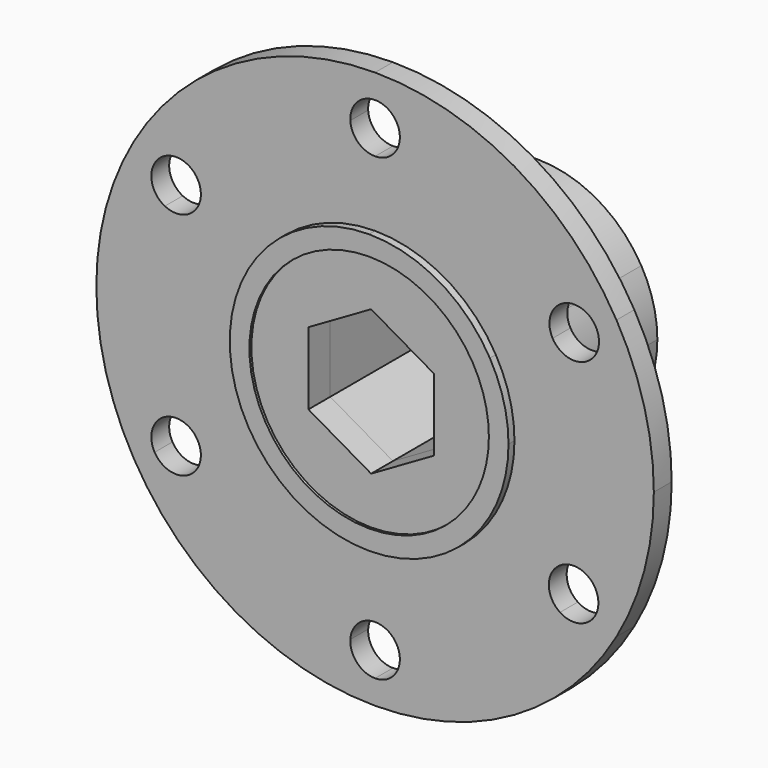
from build123d import *

# Parameters (mm, degrees)
F1_DEPTH = 18.542
F2_DEPTH = 3.048
F3_DEPTH = 2.286
F4_DEPTH = 2.286
F6_DEPTH = 2.794


# Not quite as in the source:
# - a feature of the source that left no trace in its solid (it failed there, or was rolled back) is left out


with BuildPart() as f1:
    # F0 (on Front) → F1 (new body)
    with BuildSketch(Plane.XZ):
        with BuildLine():
            Line((6.4262, 3.7101682999), (10.6292995539, 6.1368289587))
            ThreePointArc((10.6292995539, 6.1368289587), (6.1368289587, 10.6292995539), (0, 12.2736579174))
            Line((0, 12.2736579174), (0, 7.4203365997))
            Line((0, 7.4203365997), (6.4262, 3.7101682999))
        make_face()
        with BuildLine():
            ThreePointArc((12.2736579174, 0), (11.8554431655, 3.1766564221), (10.6292995539, 6.1368289587))
            Line((10.6292995539, 6.1368289587), (6.4262, 3.7101682999))
            Line((6.4262, 3.7101682999), (6.4262, -2.8670745859))
            Line((6.4262, -2.8670745859), (6.4262, -3.7101682999))
            Line((6.4262, -3.7101682999), (10.6292995539, -6.1368289587))
            ThreePointArc((10.6292995539, -6.1368289587), (11.8554431655, -3.1766564221), (12.2736579174, 0))
        make_face()
        with BuildLine():
            ThreePointArc((0, -12.2736579174), (6.1368289587, -10.6292995539), (10.6292995539, -6.1368289587))
            Line((10.6292995539, -6.1368289587), (6.4262, -3.7101682999))
            Line((6.4262, -3.7101682999), (0, -7.4203365997))
            Line((0, -7.4203365997), (0, -12.2736579174))
        make_face()
        with BuildLine():
            Line((0, 7.4203365997), (0, 12.2736579174))
            ThreePointArc((0, 12.2736579174), (-6.1368289587, 10.6292995539), (-10.6292995539, 6.1368289587))
            Line((-10.6292995539, 6.1368289587), (-6.4262, 3.7101682999))
            Line((-6.4262, 3.7101682999), (0, 7.4203365997))
        make_face()
        with BuildLine():
            ThreePointArc((-10.6292995539, -6.1368289587), (-6.1368289587, -10.6292995539), (0, -12.2736579174))
            Line((0, -12.2736579174), (0, -7.4203365997))
            Line((0, -7.4203365997), (-6.4262, -3.7101682999))
            Line((-6.4262, -3.7101682999), (-10.6292995539, -6.1368289587))
        make_face()
        with BuildLine():
            Line((-6.4262, 3.7101682999), (-10.6292995539, 6.1368289587))
            ThreePointArc((-10.6292995539, 6.1368289587), (-12.2736579174, 0), (-10.6292995539, -6.1368289587))
            Line((-10.6292995539, -6.1368289587), (-6.4262, -3.7101682999))
            Line((-6.4262, -3.7101682999), (-6.4262, 3.7101682999))
        make_face()
    extrude(amount=-F1_DEPTH)

    # F0 (on Front) → F6 (join)
    with BuildSketch(Plane.XZ):
        with BuildLine():
            Line((6.4262, 3.7101682999), (10.6292995539, 6.1368289587))
            ThreePointArc((10.6292995539, 6.1368289587), (6.1368289587, 10.6292995539), (0, 12.2736579174))
            Line((0, 12.2736579174), (0, 7.4203365997))
            Line((0, 7.4203365997), (6.4262, 3.7101682999))
        make_face()
        with BuildLine():
            ThreePointArc((12.2736579174, 0), (11.8554431655, 3.1766564221), (10.6292995539, 6.1368289587))
            Line((10.6292995539, 6.1368289587), (6.4262, 3.7101682999))
            Line((6.4262, 3.7101682999), (6.4262, -2.8670745859))
            Line((6.4262, -2.8670745859), (6.4262, -3.7101682999))
            Line((6.4262, -3.7101682999), (10.6292995539, -6.1368289587))
            ThreePointArc((10.6292995539, -6.1368289587), (11.8554431655, -3.1766564221), (12.2736579174, 0))
        make_face()
        with BuildLine():
            ThreePointArc((0, -12.2736579174), (6.1368289587, -10.6292995539), (10.6292995539, -6.1368289587))
            Line((10.6292995539, -6.1368289587), (6.4262, -3.7101682999))
            Line((6.4262, -3.7101682999), (0, -7.4203365997))
            Line((0, -7.4203365997), (0, -12.2736579174))
        make_face()
        with BuildLine():
            Line((0, 7.4203365997), (0, 12.2736579174))
            ThreePointArc((0, 12.2736579174), (-6.1368289587, 10.6292995539), (-10.6292995539, 6.1368289587))
            Line((-10.6292995539, 6.1368289587), (-6.4262, 3.7101682999))
            Line((-6.4262, 3.7101682999), (0, 7.4203365997))
        make_face()
        with BuildLine():
            ThreePointArc((-10.6292995539, -6.1368289587), (-6.1368289587, -10.6292995539), (0, -12.2736579174))
            Line((0, -12.2736579174), (0, -7.4203365997))
            Line((0, -7.4203365997), (-6.4262, -3.7101682999))
            Line((-6.4262, -3.7101682999), (-10.6292995539, -6.1368289587))
        make_face()
        with BuildLine():
            Line((-6.4262, 3.7101682999), (-10.6292995539, 6.1368289587))
            ThreePointArc((-10.6292995539, 6.1368289587), (-12.2736579174, 0), (-10.6292995539, -6.1368289587))
            Line((-10.6292995539, -6.1368289587), (-6.4262, -3.7101682999))
            Line((-6.4262, -3.7101682999), (-6.4262, 3.7101682999))
        make_face()
    extrude(amount=F6_DEPTH)


with BuildPart() as f2:
    # F0 (on Front) → F2 (new body)
    with BuildSketch(Plane.XZ):
        with BuildLine():
            ThreePointArc((0, -14.2875), (7.14375, -12.3733379566), (12.3733379566, -7.14375))
            Line((12.3733379566, -7.14375), (10.6292995539, -6.1368289587))
            ThreePointArc((10.6292995539, -6.1368289587), (6.1368289587, -10.6292995539), (0, -12.2736579174))
            Line((0, -12.2736579174), (0, -14.2875))
        make_face()
        with BuildLine():
            ThreePointArc((-12.3733379566, -7.14375), (-7.14375, -12.3733379566), (0, -14.2875))
            Line((0, -14.2875), (0, -12.2736579174))
            ThreePointArc((0, -12.2736579174), (-6.1368289587, -10.6292995539), (-10.6292995539, -6.1368289587))
            Line((-10.6292995539, -6.1368289587), (-12.3733379566, -7.14375))
        make_face()
        with BuildLine():
            Line((-10.6292995539, 6.1368289587), (-12.3733379566, 7.14375))
            ThreePointArc((-12.3733379566, 7.14375), (-14.2875, 0), (-12.3733379566, -7.14375))
            Line((-12.3733379566, -7.14375), (-10.6292995539, -6.1368289587))
            ThreePointArc((-10.6292995539, -6.1368289587), (-12.2736579174, 0), (-10.6292995539, 6.1368289587))
        make_face()
        with BuildLine():
            Line((0, 12.2736579174), (0, 14.2875))
            ThreePointArc((0, 14.2875), (-7.14375, 12.3733379566), (-12.3733379566, 7.14375))
            Line((-12.3733379566, 7.14375), (-10.6292995539, 6.1368289587))
            ThreePointArc((-10.6292995539, 6.1368289587), (-6.1368289587, 10.6292995539), (0, 12.2736579174))
        make_face()
        with BuildLine():
            Line((10.6292995539, 6.1368289587), (12.3733379566, 7.14375))
            ThreePointArc((12.3733379566, 7.14375), (7.14375, 12.3733379566), (0, 14.2875))
            Line((0, 14.2875), (0, 12.2736579174))
            ThreePointArc((0, 12.2736579174), (6.1368289587, 10.6292995539), (10.6292995539, 6.1368289587))
        make_face()
        with BuildLine():
            ThreePointArc((14.2875, 0), (13.8006652431, 3.6978771069), (12.3733379566, 7.14375))
            Line((12.3733379566, 7.14375), (10.6292995539, 6.1368289587))
            ThreePointArc((10.6292995539, 6.1368289587), (11.8554431655, 3.1766564221), (12.2736579174, 0))
            ThreePointArc((12.2736579174, 0), (11.8554431655, -3.1766564221), (10.6292995539, -6.1368289587))
            Line((10.6292995539, -6.1368289587), (12.3733379566, -7.14375))
            ThreePointArc((12.3733379566, -7.14375), (13.8006652431, -3.6978771069), (14.2875, 0))
        make_face()
    extrude(amount=F2_DEPTH)

    # F0 (on Front) → F3 (join)
    with BuildSketch(Plane.XZ):
        with BuildLine():
            ThreePointArc((2.5363048132, -23.415995125), (11.7362040327, -20.4206558343), (18.9556707318, -13.9794211936))
            ThreePointArc((18.9556707318, -13.9794211936), (17.8690577157, -12.3976727234), (18.1990671233, -10.5072363026))
            Line((18.1990671233, -10.5072363026), (12.3733379566, -7.14375))
            ThreePointArc((12.3733379566, -7.14375), (7.14375, -12.3733379566), (0, -14.2875))
            Line((0, -14.2875), (0, -21.0129545875))
            ThreePointArc((0, -21.0129545875), (1.7469577793, -21.7091166019), (2.5363048132, -23.415995125))
        make_face()
        with BuildLine():
            ThreePointArc((-19.0106942266, -13.9045019625), (-11.7764772938, -20.397457007), (-2.5363048132, -23.415995125))
            ThreePointArc((-2.5363048132, -23.415995125), (-1.7469577793, -21.7091166019), (0, -21.0129545875))
            Line((0, -21.0129545875), (0, -14.2875))
            ThreePointArc((0, -14.2875), (-7.14375, -12.3733379566), (-12.3733379566, -7.14375))
            Line((-12.3733379566, -7.14375), (-18.1977524814, -10.5064772938))
            ThreePointArc((-18.1977524814, -10.5064772938), (-17.9440054082, -11.1190769192), (-17.857457007, -11.7764772938))
            ThreePointArc((-17.857457007, -11.7764772938), (-18.1643003329, -12.9866885434), (-19.0106942266, -13.9045019625))
        make_face()
        with BuildLine():
            ThreePointArc((-18.1977524814, 10.5064772938), (-19.6741253606, 9.3416484847), (-21.5469990398, 9.5114931625))
            ThreePointArc((-21.5469990398, 9.5114931625), (-23.5529545875, 0), (-21.5469990398, -9.5114931625))
            ThreePointArc((-21.5469990398, -9.5114931625), (-19.6741253606, -9.3416484847), (-18.1977524814, -10.5064772938))
            Line((-18.1977524814, -10.5064772938), (-12.3733379566, -7.14375))
            ThreePointArc((-12.3733379566, -7.14375), (-14.2875, 0), (-12.3733379566, 7.14375))
            Line((-12.3733379566, 7.14375), (-18.1977524814, 10.5064772938))
        make_face()
        with BuildLine():
            ThreePointArc((0, 21.0129545875), (-1.7469577793, 21.7091166019), (-2.5363048132, 23.415995125))
            ThreePointArc((-2.5363048132, 23.415995125), (-11.7764772938, 20.397457007), (-19.0106942266, 13.9045019625))
            ThreePointArc((-19.0106942266, 13.9045019625), (-18.1643003329, 12.9866885434), (-17.857457007, 11.7764772938))
            ThreePointArc((-17.857457007, 11.7764772938), (-17.9440054082, 11.1190769192), (-18.1977524814, 10.5064772938))
            Line((-18.1977524814, 10.5064772938), (-12.3733379566, 7.14375))
            ThreePointArc((-12.3733379566, 7.14375), (-7.14375, 12.3733379566), (0, 14.2875))
            Line((0, 14.2875), (0, 21.0129545875))
        make_face()
        with BuildLine():
            ThreePointArc((18.1979169714, 10.5065722621), (17.9478924637, 12.356678067), (19.0300897095, 13.8779449289))
            ThreePointArc((19.0300897095, 13.8779449289), (11.790714294, 20.3892306436), (2.5363048132, 23.415995125))
            ThreePointArc((2.5363048132, 23.415995125), (1.7469577793, 21.7091166019), (0, 21.0129545875))
            Line((0, 21.0129545875), (0, 14.2875))
            ThreePointArc((0, 14.2875), (7.14375, 12.3733379566), (12.3733379566, 7.14375))
            Line((12.3733379566, 7.14375), (18.1979169714, 10.5065722621))
        make_face()
        with BuildLine():
            ThreePointArc((23.5529545875, 0), (23.0493975606, 4.8442689742), (21.5602583585, 9.4813991223))
            ThreePointArc((21.5602583585, 9.4813991223), (19.6731048169, 9.3184074624), (18.1979169714, 10.5065722621))
            Line((18.1979169714, 10.5065722621), (12.3733379566, 7.14375))
            ThreePointArc((12.3733379566, 7.14375), (13.8006652431, 3.6978771069), (14.2875, 0))
            ThreePointArc((14.2875, 0), (13.8006652431, -3.6978771069), (12.3733379566, -7.14375))
            Line((12.3733379566, -7.14375), (18.1990671233, -10.5072363026))
            ThreePointArc((18.1990671233, -10.5072363026), (19.5459299692, -9.4477887138), (21.2591419094, -9.484850376))
            ThreePointArc((21.2591419094, -9.484850376), (21.3857231383, -9.5372788153), (21.5092932207, -9.5964563744))
            ThreePointArc((21.5092932207, -9.5964563744), (23.0363742399, -4.9058262996), (23.5529545875, 0))
        make_face()
    extrude(amount=F3_DEPTH)

    # F0 (on Front) → F4 (join)
    with BuildSketch(Plane.XZ):
        with BuildLine():
            Line((22.596957278, 13.0463593673), (24.7466759131, 14.2875))
            ThreePointArc((24.7466759131, 14.2875), (14.2875, 24.7466759131), (0, 28.575))
            Line((0, 28.575), (0, 26.0929545875))
            ThreePointArc((0, 26.0929545875), (1.7960512242, 25.3490058117), (2.54, 23.5529545875))
            ThreePointArc((2.54, 23.5529545875), (2.5390760353, 23.4844499366), (2.5363048132, 23.415995125))
            ThreePointArc((2.5363048132, 23.415995125), (11.790714294, 20.3892306436), (19.0300897095, 13.8779449289))
            ThreePointArc((19.0300897095, 13.8779449289), (20.9905935558, 14.2216476119), (22.596957278, 13.0463593673))
        make_face()
        with BuildLine():
            Line((0, 26.0929545875), (0, 28.575))
            ThreePointArc((0, 28.575), (-14.2875, 24.7466759131), (-24.7466759131, 14.2875))
            Line((-24.7466759131, 14.2875), (-22.5971615326, 13.0464772938))
            ThreePointArc((-22.5971615326, 13.0464772938), (-20.9884478303, 14.2467667194), (-19.0106942266, 13.9045019625))
            ThreePointArc((-19.0106942266, 13.9045019625), (-11.7764772938, 20.397457007), (-2.5363048132, 23.415995125))
            ThreePointArc((-2.5363048132, 23.415995125), (-1.8438379857, 25.2999123668), (0, 26.0929545875))
        make_face()
        with BuildLine():
            Line((-22.5971615326, 13.0464772938), (-24.7466759131, 14.2875))
            ThreePointArc((-24.7466759131, 14.2875), (-28.575, 0), (-24.7466759131, -14.2875))
            Line((-24.7466759131, -14.2875), (-22.5971615326, -13.0464772938))
            ThreePointArc((-22.5971615326, -13.0464772938), (-22.832285816, -11.0531456474), (-21.5469990398, -9.5114931625))
            ThreePointArc((-21.5469990398, -9.5114931625), (-23.5529545875, 0), (-21.5469990398, 9.5114931625))
            ThreePointArc((-21.5469990398, 9.5114931625), (-22.832285816, 11.0531456474), (-22.5971615326, 13.0464772938))
        make_face()
        with BuildLine():
            ThreePointArc((-24.7466759131, -14.2875), (-14.2875, -24.7466759131), (0, -28.575))
            Line((0, -28.575), (0, -26.0929545875))
            ThreePointArc((0, -26.0929545875), (-1.8438379857, -25.2999123668), (-2.5363048132, -23.415995125))
            ThreePointArc((-2.5363048132, -23.415995125), (-11.7764772938, -20.397457007), (-19.0106942266, -13.9045019625))
            ThreePointArc((-19.0106942266, -13.9045019625), (-20.9884478303, -14.2467667194), (-22.5971615326, -13.0464772938))
            Line((-22.5971615326, -13.0464772938), (-24.7466759131, -14.2875))
        make_face()
        with BuildLine():
            ThreePointArc((0, -28.575), (14.2875, -24.7466759131), (24.7466759131, -14.2875))
            Line((24.7466759131, -14.2875), (22.5955291864, -13.0455348583))
            ThreePointArc((22.5955291864, -13.0455348583), (20.9820683001, -14.3171964463), (18.9556707318, -13.9794211936))
            ThreePointArc((18.9556707318, -13.9794211936), (11.7362040327, -20.4206558343), (2.5363048132, -23.415995125))
            ThreePointArc((2.5363048132, -23.415995125), (2.5390760353, -23.4844499366), (2.54, -23.5529545875))
            ThreePointArc((2.54, -23.5529545875), (1.7960512242, -25.3490058117), (0, -26.0929545875))
            Line((0, -26.0929545875), (0, -28.575))
        make_face()
        with BuildLine():
            ThreePointArc((24.7466759131, -14.2875), (27.6013304862, -7.3957542138), (28.575, 0))
            ThreePointArc((28.575, 0), (27.6013304862, 7.3957542138), (24.7466759131, 14.2875))
            Line((24.7466759131, 14.2875), (22.596957278, 13.0463593673))
            ThreePointArc((22.596957278, 13.0463593673), (22.8630243002, 12.4212555209), (22.9538799063, 11.7479860816))
            ThreePointArc((22.9538799063, 11.7479860816), (22.5776036951, 10.4176104333), (21.5602583585, 9.4813991223))
            ThreePointArc((21.5602583585, 9.4813991223), (23.0493975606, 4.8442689742), (23.5529545875, 0))
            ThreePointArc((23.5529545875, 0), (23.0363742399, -4.9058262996), (21.5092932207, -9.5964563744))
            ThreePointArc((21.5092932207, -9.5964563744), (22.5180912242, -10.5322954019), (22.8908211645, -11.8568860891))
            ThreePointArc((22.8908211645, -11.8568860891), (22.8158930069, -12.4692755176), (22.5955291864, -13.0455348583))
            Line((22.5955291864, -13.0455348583), (24.7466759131, -14.2875))
        make_face()
    extrude(amount=F4_DEPTH)


solid = Compound([f1.part, f2.part])
